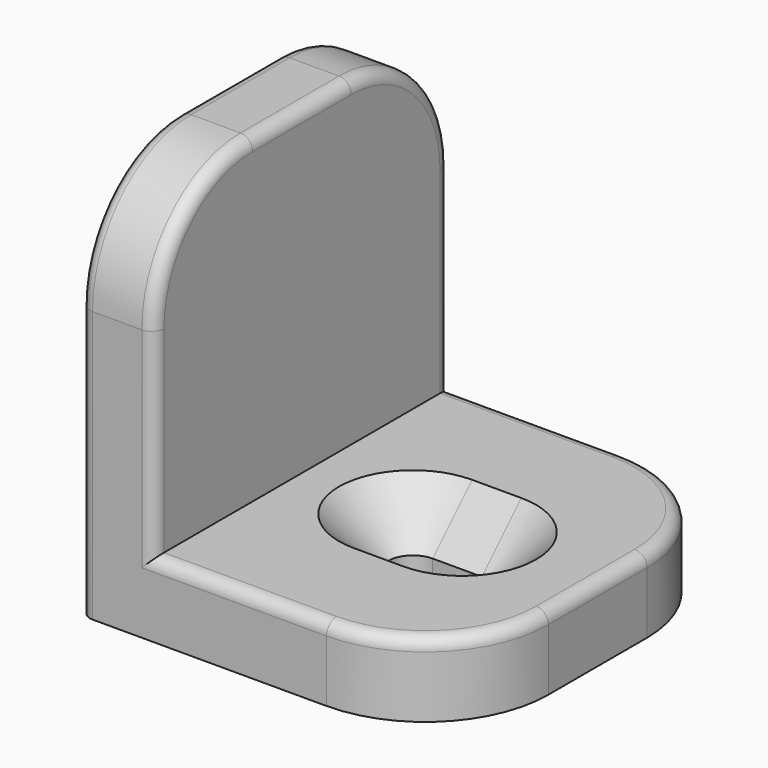
from build123d import *

# Parameters (mm, degrees)
F0_W     = 3
F0_H     = 15
F1_DEPTH = 16
F0_W_2   = 12
F2_DEPTH = 3
F3_R     = 5.5
F4_DEPTH = 1
F5_SIZE  = 2
F6_R     = 5
F7_R     = 0.5


with BuildPart() as f1:
    # F0 (on Top) → F1 (new body)
    with BuildSketch(Plane.XY):
        with Locations((-6, 0)):
            Rectangle(F0_W, F0_H)
    extrude(amount=F1_DEPTH)

    # F0 (on Top) → F2 (join)
    with BuildSketch(Plane.XY):
        with Locations((1.5, 0)):
            Rectangle(F0_W_2, F0_H)
        with BuildLine():
            ThreePointArc((0, -1), (-1, 0), (0, 1))
            Line((0, 1), (2, 1))
            ThreePointArc((2, 1), (2.7071067812, 0.7071067812), (3, 0))
            ThreePointArc((3, 0), (2.7071067812, -0.7071067812), (2, -1))
            Line((2, -1), (0, -1))
        make_face(mode=Mode.SUBTRACT)
    extrude(amount=F2_DEPTH)

    # F3 (on face) → F4 (cut)
    with BuildSketch(Plane(origin=(-7.5, 0, 0), x_dir=(0, -1, 0), z_dir=(-1, 0, 0))):
        with Locations((0, 8)):
            Circle(F3_R)
    extrude(amount=-F4_DEPTH, mode=Mode.SUBTRACT)

    # F5
    f5_edges = [f1.edges().sort_by_distance(p)[0] for p in [
        (-1, 0, 3),
    ]]
    chamfer(f5_edges, length=F5_SIZE)

    # F6
    f6_edges = [f1.edges().sort_by_distance(p)[0] for p in [
        (-6, -7.5, 16),
        (-6, 7.5, 16),
        (7.5, -7.5, 1.5),
        (7.5, 7.5, 1.5),
    ]]
    fillet(f6_edges, radius=F6_R)

    # F7
    f7_edges = [f1.edges().sort_by_distance(p)[0] for p in [
        (-7.5, 5.5, 8),
        (-7.5, 6.035534, 14.535534),
        (-4.5, -6.035534, 14.535534),
        (6.035534, -6.035534, 3),
    ]]
    fillet(f7_edges, radius=F7_R)


solid = f1.part
